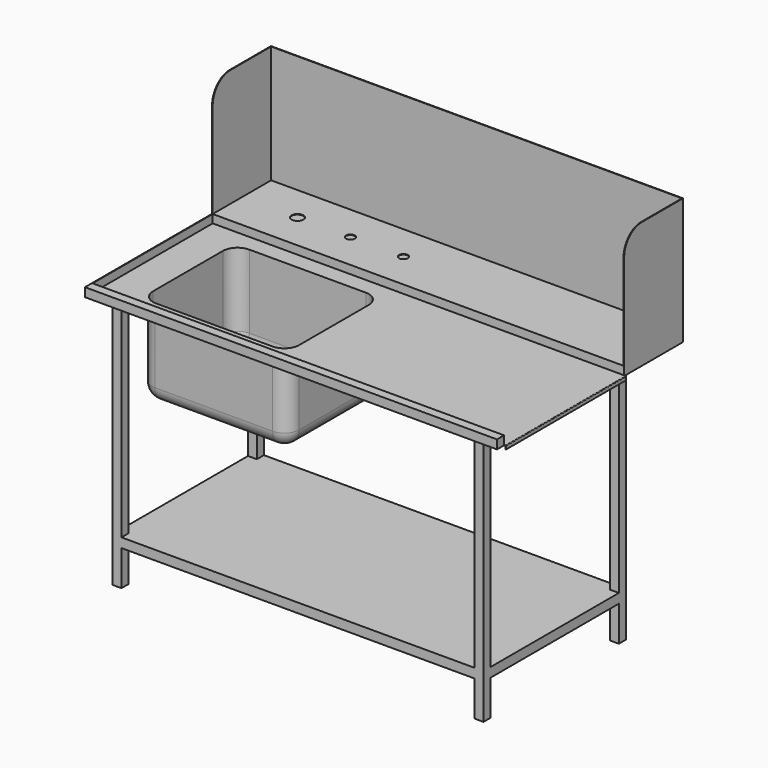
from build123d import *

# Parameters (mm, degrees)
F0_W        = 1400
F0_H        = 790
F1_DEPTH    = 30
F2_W        = 1398
F2_H        = 510
F3_DEPTH    = 28
F4_W        = 500
F4_H        = 400
F5_DEPTH    = 300
F6_T        = 2
F6_T3_DEPTH = 404
F6_T5_DEPTH = 504
F6_T7_DEPTH = 32
F7_R        = 50
F8_R        = 25
F9_DEPTH    = 2
F10_R       = 15
F10_R_2     = 20
F11_DEPTH   = 30
F12_W       = 510
F12_H       = 2
F13_DEPTH   = 5
F14_W       = 510
F14_H       = 2
F15_ANGLE   = 90
F16_W       = 2
F16_H       = 510
F17_DEPTH   = 10
F18_W       = 30
F18_H       = 30
F19_DEPTH   = 850
F20_W       = 30
F20_H       = 30
F21_DEPTH   = 1200
F22_W       = 30
F22_H       = 30
F23_DEPTH   = 545
F25_DEPTH   = 2
F27_DEPTH   = 400
F28_R       = 75


# Not quite as in the source:
# - a shell that OpenCascade refuses in one call is made with other operations: the cavity is built on its own and cut out


with BuildPart() as f1:
    # F0 (on Top) → F1 (new body)
    with BuildSketch(Plane.XY):
        with Locations((700, 395)):
            Rectangle(F0_W, F0_H)
    extrude(amount=F1_DEPTH)

    # F2 (on face) → F3 (cut)
    with BuildSketch(Plane.XY.offset(30)):
        with Locations((701, 285)):
            Rectangle(F2_W, F2_H)
    extrude(amount=-F3_DEPTH, mode=Mode.SUBTRACT)

    # F4 (on face) → F5 (join)
    with BuildSketch(Plane(origin=(0, 0, 0), x_dir=(1, 0, 0), z_dir=(0, 0, -1))):
        with Locations((370, -285)):
            Rectangle(F4_W, F4_H)
    extrude(amount=F5_DEPTH)

    # F6: shell of thickness 2, made by hand


with BuildPart() as f6_core1:
    # F6_t2: copy of F1
    add(f1.part)

    # the walls: a layer under each face that stays
    f6_faces = [f6_core1.faces().sort_by_distance(p)[0] for p in [
        (0, 395, 15),
        (700, 790, 15),
        (700, 0, 15),
        (700, 395, 0),
        (233.3333333333, 658.3333333333, 30),
        (1400, 658.3333333333, 25),
        (620, 285, -150),
        (370, 485, -150),
        (120, 285, -150),
        (370, 85, -150),
        (701, 540, 16),
        (2, 285, 16),
        (701, 30, 16),
        (370, 285, -300),
    ]]
    thicken(f6_faces, amount=-F6_T, mode=Mode.SUBTRACT)

    # F6_s4 → F6_t3 (cut)
    with BuildSketch(Plane.XZ.offset(-487)):
        Polygon((620.02, -0.02), (620, 2), (618, 2), (618, 0), align=None)
        Polygon((119.98, -0.02), (120, 2), (122, 2), (122, 0), align=None)
    extrude(amount=F6_T3_DEPTH, mode=Mode.SUBTRACT)

    # F6_s6 → F6_t5 (cut)
    with BuildSketch(Plane.YZ.offset(118)):
        Polygon((485.02, -0.02), (485, 2), (483, 2), (483, 0), align=None)
        Polygon((84.98, -0.02), (85, 2), (87, 2), (87, 0), align=None)
    extrude(amount=F6_T5_DEPTH, mode=Mode.SUBTRACT)

    # F6_s8 → F6_t7 (cut)
    with BuildSketch(Plane.XY):
        Polygon((2.02, 539.98), (2, 542), (0, 542), (0, 540), align=None)
        Polygon((2.02, 30.02), (0, 30), (0, 28), (2, 28), align=None)
    extrude(amount=F6_T7_DEPTH, mode=Mode.SUBTRACT)


with BuildPart() as f1_1:
    add(f1.part)

    # what is left inside the walls is the cavity
    f6_cavity = [f6_core1.part.solids().sort_by_distance(p)[0] for p in [
        (700, 10.666667, 2.02),
        (700, 624, 27.98),
        (370, 351, -297.98),
    ]]
    add(f6_cavity, mode=Mode.SUBTRACT)

    # F7
    f7_edges = [f1_1.edges().sort_by_distance(p)[0] for p in [
        (122, 483, -148),
        (618, 483, -148),
        (122, 87, -148),
        (618, 87, -148),
        (618, 285, -298),
        (370, 483, -298),
        (122, 285, -298),
        (370, 87, -298),
        (120, 85, -150),
        (370, 85, -300),
        (620, 85, -150),
        (620, 285, -300),
        (620, 485, -150),
        (370, 485, -300),
        (120, 485, -150),
        (120, 285, -300),
    ]]
    fillet(f7_edges, radius=F7_R)

    # F8 (on face) → F9 (cut, through all)
    with BuildSketch(Plane.XY.offset(-298)):
        with Locations((488, 353)):
            Circle(F8_R)
    extrude(amount=-F9_DEPTH, mode=Mode.SUBTRACT)

    # F10 (on face) → F11 (cut, through all)
    with BuildSketch(Plane.XY.offset(30)):
        with Locations((550, 665)):
            Circle(F10_R)
        with Locations((370, 665)):
            Circle(F10_R)
        with Locations((190, 665)):
            Circle(F10_R_2)
    extrude(amount=-F11_DEPTH, mode=Mode.SUBTRACT)

    # F12 (on face) → F13 (join)
    with BuildSketch(Plane.YZ.offset(1400)):
        with Locations((285, 1)):
            Rectangle(F12_W, F12_H)
    extrude(amount=F13_DEPTH)

    # F14 (on face) → F15 (revolve)
    with BuildSketch(Plane.YZ.offset(1405)):
        with Locations((285, 1)):
            Rectangle(F14_W, F14_H)
    revolve(axis=Axis((1405, 285, 0), (0, 1, 0)), revolution_arc=F15_ANGLE)

    # F16 (on face) → F17 (join)
    with BuildSketch(Plane(origin=(0, 0, 0), x_dir=(1, 0, 0), z_dir=(0, 0, -1))):
        with Locations((1406, -285)):
            Rectangle(F16_W, F16_H)
    extrude(amount=F17_DEPTH)

    # F18 (on face) → F19 (join)
    with BuildSketch(Plane(origin=(0, 0, 0), x_dir=(1, 0, 0), z_dir=(0, 0, -1))):
        with Locations((85, -45)):
            Rectangle(F18_W, F18_H)
        with Locations((1315, -45)):
            Rectangle(F18_W, F18_H)
        with Locations((1315, -620)):
            Rectangle(F18_W, F18_H)
        with Locations((85, -620)):
            Rectangle(F18_W, F18_H)
    extrude(amount=F19_DEPTH)

    # F20 (on face) → F21 (join, through all)
    with BuildSketch(Plane.YZ.offset(100)):
        with Locations((45, -715)):
            Rectangle(F20_W, F20_H)
        with Locations((620, -715)):
            Rectangle(F20_W, F20_H)
    extrude(amount=F21_DEPTH)

    # F22 (on face) → F23 (join, through all)
    with BuildSketch(Plane(origin=(0, 60, 0), x_dir=(-1, 0, 0), z_dir=(0, 1, 0))):
        with Locations((-1315, -715)):
            Rectangle(F22_W, F22_H)
        with Locations((-85, -715)):
            Rectangle(F22_W, F22_H)
    extrude(amount=F23_DEPTH)

    # F24 (on face) → F25 (join)
    with BuildSketch(Plane.XY.offset(-700)):
        Polygon((100, 60), (100, 30), (1300, 30), (1300, 60), (1330, 60), (1330, 605), (1300, 605), (1300, 635), (100, 635), (100, 605), (70, 605), (70, 60), align=None)
    extrude(amount=F25_DEPTH)

    # F26 (on face) → F27 (join)
    with BuildSketch(Plane.XY.offset(30)):
        Polygon((1400, 790), (0, 790), (0, 540), (2, 540), (2, 788), (1398, 788), (1398, 540), (1400, 540), align=None)
    extrude(amount=F27_DEPTH)

    # F28
    f28_edges = [f1_1.edges().sort_by_distance(p)[0] for p in [
        (1, 540, 430),
        (1399, 540, 430),
    ]]
    fillet(f28_edges, radius=F28_R)


solid = f1_1.part
